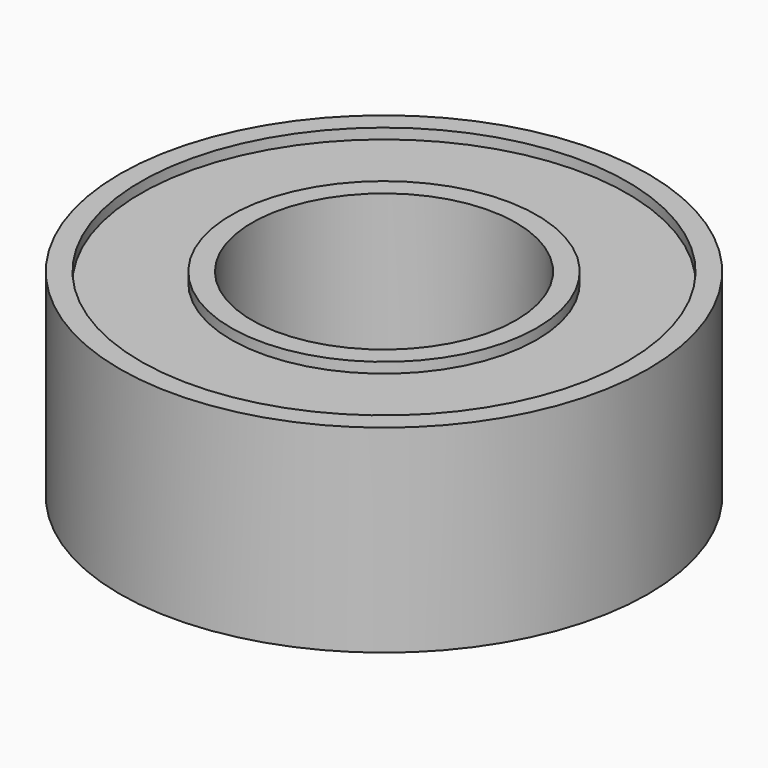
from build123d import *

# Parameters (mm, degrees)
F0_R     = 3.675
F0_R_2   = 3.175
F1_DEPTH = 2.38125
F0_R_3   = 6.35
F0_R_4   = 5.85
F3_R     = 5.85
F3_R_2   = 3.675
F4_DEPTH = 0.25


# Not quite as in the source:
# - a length typed as a fraction of an inch, garbled in the dataset ("3 / 203.2 mm" for 3/8 in), is restored


with BuildPart() as f1:
    # F0 (on Top) → F1 (new body, symmetric)
    with BuildSketch(Plane.XY):
        Circle(F0_R)
        Circle(F0_R_2, mode=Mode.SUBTRACT)
    extrude(amount=F1_DEPTH, both=True)



with BuildPart() as f1b:
    # F0 (on Top) → F1, piece 2 (new body, symmetric)
    with BuildSketch(Plane.XY):
        Circle(F0_R_3)
        Circle(F0_R_4, mode=Mode.SUBTRACT)
    extrude(amount=F1_DEPTH, both=True)


with BuildPart() as f1_1:
    add(f1.part)

    add(f1b.part)  # F4 merges F1b
    # F3 (on offset) → F4 (join)
    with BuildSketch(Plane.XY.offset(1.88125)):
        Circle(F3_R)
        Circle(F3_R_2, mode=Mode.SUBTRACT)
    extrude(amount=F4_DEPTH)

    # F5: F1 across plane


with BuildPart() as f1_2:
    add(f1_1.part)
    add(f1_1.part.mirror(Plane.XY))


solid = f1_2.part
